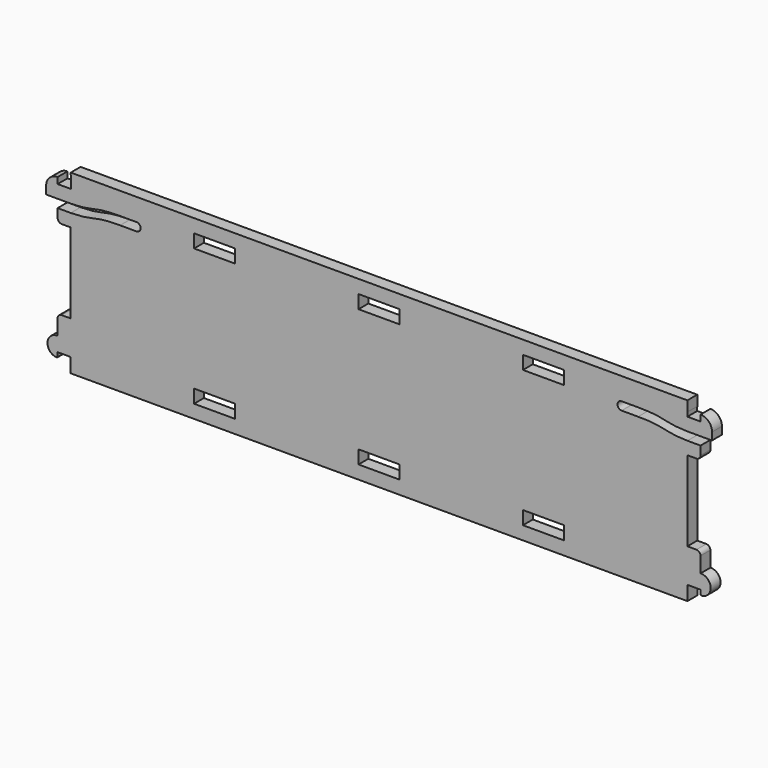
from build123d import *

# Parameters (mm, degrees)
F0_W     = 10
F0_H     = 3.25
F1_DEPTH = 3


# Not quite as in the source:
# - ends of sketch curves that miss each other by under 0.0002 mm in the source are joined


with BuildPart() as f1:
    # F0 (on Front) → F1 (new body)
    with BuildSketch(Plane.XZ):
        with BuildLine():
            Line((75, 21.5), (-75, 21.5))
            Line((-75, 21.5), (-74.9930354723, 18.0000069292))
            Line((-74.9930354723, 18.0000069292), (-78.2, 18.0000069292))
            Line((-78.2, 18.0000069292), (-78.2, 19.5000069292))
            ThreePointArc((-78.2, 19.5000069292), (-80.1867814364, 18.6729994594), (-80.999932095, 16.6805065893))
            Line((-80.999932095, 16.6805065893), (-80.9871833927, 14.85))
            Line((-80.9871833927, 14.85), (-75.0000029802, 14.85))
            add(Edge.make_bspline(
                [(-75.0000029802, 14.85), (-72.0000029802, 14.85), (-69.0064407929, 15.7236590768), (-66.0000029802, 16.1), (-63.0000029802, 16.1)],
                knots=[0, 0, 0, 0, 0.5005364838, 1, 1, 1, 1], degree=3))
            Line((-63.0000029802, 16.1), (-59.0000029802, 16.1))
            ThreePointArc((-59.0000029802, 16.1), (-58.0000029802, 15.1), (-59.0000029802, 14.1))
            Line((-59.0000029802, 14.1), (-63.0000029802, 14.1))
            add(Edge.make_bspline(
                [(-74.9999980132, 12.85), (-71.9999980132, 12.85), (-69.0064358259, 13.7236590768), (-65.9999980132, 14.1), (-63.0000029802, 14.1)],
                knots=[0, 0, 0, 0, 0.5005364838, 1, 1, 1, 1], degree=3))
            Line((-74.9999980132, 12.85), (-78.2, 12.85))
            Line((-78.2, 12.85), (-78.2, 10.75))
            ThreePointArc((-78.2, 10.75), (-77.9071067812, 10.0428932188), (-77.2, 9.75))
            Line((-77.2, 9.75), (-75, 9.75))
            Line((-75, 9.75), (-75, -9.75))
            Line((-75, -9.75), (-75, -18.0000069292))
            Line((-75, -18.0000069292), (-75, -21.5))
            Line((-75, -21.5), (75, -21.5))
            Line((75, -21.5), (75, -18.0000069292))
            Line((75, -18.0000069292), (75, -9.75))
            Line((75, -9.75), (75, 9.75))
            Line((75, 9.75), (77.2, 9.75))
            ThreePointArc((77.2, 9.75), (77.9071067812, 10.0428932188), (78.2, 10.75))
            Line((78.2, 10.75), (78.2, 12.85))
            Line((78.2, 12.85), (74.9999980132, 12.85))
            add(Edge.make_bspline(
                [(74.9999980132, 12.85), (71.9999980132, 12.85), (69.0064358259, 13.7236590768), (65.9999980132, 14.1), (62.9999980132, 14.1)],
                knots=[0, 0, 0, 0, 0.5005364838, 1, 1, 1, 1], degree=3))
            Line((62.9999980132, 14.1), (59.0000029802, 14.1))
            ThreePointArc((59.0000029802, 14.1), (58.0000029802, 15.1), (59.0000029802, 16.1))
            Line((59.0000029802, 16.1), (63.0000029802, 16.1))
            add(Edge.make_bspline(
                [(74.9710970223, 14.8500135578), (71.9903624817, 14.8528122415), (69.001599828, 15.7242650608), (66.0000029802, 16.1), (63.0000029802, 16.1)],
                knots=[0.0016101996, 0.0016101996, 0.0016101996, 0.0016101996, 0.5005364838, 1, 1, 1, 1], degree=3))
            Line((74.9710970223, 14.8500135578), (75.0000029802, 14.85))
            Line((75.0000029802, 14.85), (80.9871833927, 14.85))
            Line((80.9871833927, 14.85), (80.999932095, 16.6805065893))
            ThreePointArc((80.999932095, 16.6805065893), (80.1867814364, 18.6729994594), (78.2, 19.5000069292))
            Line((78.2, 19.5000069292), (78.2, 18.0000069292))
            Line((78.2, 18.0000069292), (74.9930354723, 18.0000069292))
            Line((74.9930354723, 18.0000069292), (75, 19))
            Line((75, 19), (75, 21.5))
        make_face()
        with Locations((-40, -16.625)):
            Rectangle(F0_W, F0_H, mode=Mode.SUBTRACT)
        with Locations((0, -16.625)):
            Rectangle(F0_W, F0_H, mode=Mode.SUBTRACT)
        with Locations((40, -16.625)):
            Rectangle(F0_W, F0_H, mode=Mode.SUBTRACT)
        with Locations((-40, 16.625)):
            Rectangle(F0_W, F0_H, mode=Mode.SUBTRACT)
        with Locations((0, 16.625)):
            Rectangle(F0_W, F0_H, mode=Mode.SUBTRACT)
        with Locations((40, 16.625)):
            Rectangle(F0_W, F0_H, mode=Mode.SUBTRACT)
        with BuildLine():
            Line((-75, -18.0000069292), (-75, -9.75))
            Line((-75, -9.75), (-77.2, -9.75))
            ThreePointArc((-77.2, -9.75), (-77.9071067812, -10.0428932188), (-78.2, -10.75))
            Line((-78.2, -10.75), (-78.2, -12.384363041))
            Line((-78.2, -12.384363041), (-78.2, -14.5073579624))
            ThreePointArc((-78.2, -14.5073579624), (-80.6617701682, -16.7497231552), (-78.4079163074, -19.2009793215))
            ThreePointArc((-78.4079163074, -19.2009793215), (-78.2614057387, -19.1453290857), (-78.2, -19.0011360528))
            Line((-78.2, -19.0011360528), (-78.2, -18.0000069292))
            Line((-78.2, -18.0000069292), (-75, -18.0000069292))
        make_face()
        with BuildLine():
            Line((77.2, -9.75), (75, -9.75))
            Line((75, -9.75), (75, -18.0000069292))
            Line((75, -18.0000069292), (78.2, -18.0000069292))
            Line((78.2, -18.0000069292), (78.2, -19.0011360528))
            ThreePointArc((78.2, -19.0011360528), (78.2614057387, -19.1453290857), (78.4079163074, -19.2009793215))
            ThreePointArc((78.4079163074, -19.2009793215), (80.6617701682, -16.7497231552), (78.2, -14.5073579624))
            Line((78.2, -14.5073579624), (78.2, -12.384363041))
            Line((78.2, -12.384363041), (78.2, -10.75))
            ThreePointArc((78.2, -10.75), (77.9071067812, -10.0428932188), (77.2, -9.75))
        make_face()
    extrude(amount=F1_DEPTH)


solid = f1.part
